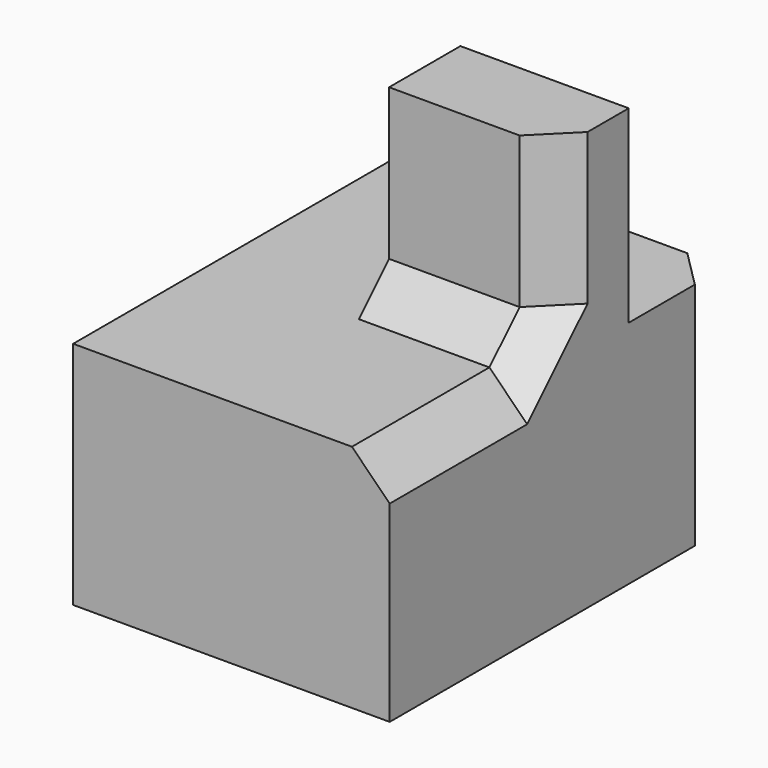
from build123d import *

# Parameters (mm, degrees)
F0_W     = 42.5828881562
F0_H     = 30.9346560389
F1_DEPTH = 56.388
F2_W     = 22.6413179189
F2_H     = 11.9935432317
F3_DEPTH = 25.4
F4_SIZE  = 5.08


with BuildPart() as f1:
    # F0 (on Front) → F1 (new body)
    with BuildSketch(Plane.XZ):
        with Locations((21.2914440781, 15.4673280194)):
            Rectangle(F0_W, F0_H)
    extrude(amount=F1_DEPTH)

    # F2 (on face) → F3 (join)
    with BuildSketch(Plane.XY.offset(30.9346560389)):
        with Locations((31.2622291967, -22.1972283841)):
            Rectangle(F2_W, F2_H)
    extrude(amount=F3_DEPTH)

    # F4
    f4_edges = [f1.edges().sort_by_distance(p)[0] for p in [
        (31.262229, -28.194, 30.934656),
        (42.582888, -42.291, 30.934656),
        (21.291444, 0, 0),
        (42.582888, 0, 15.467328),
        (42.582888, -28.194, 43.634656),
    ]]
    chamfer(f4_edges, length=F4_SIZE)


solid = f1.part
